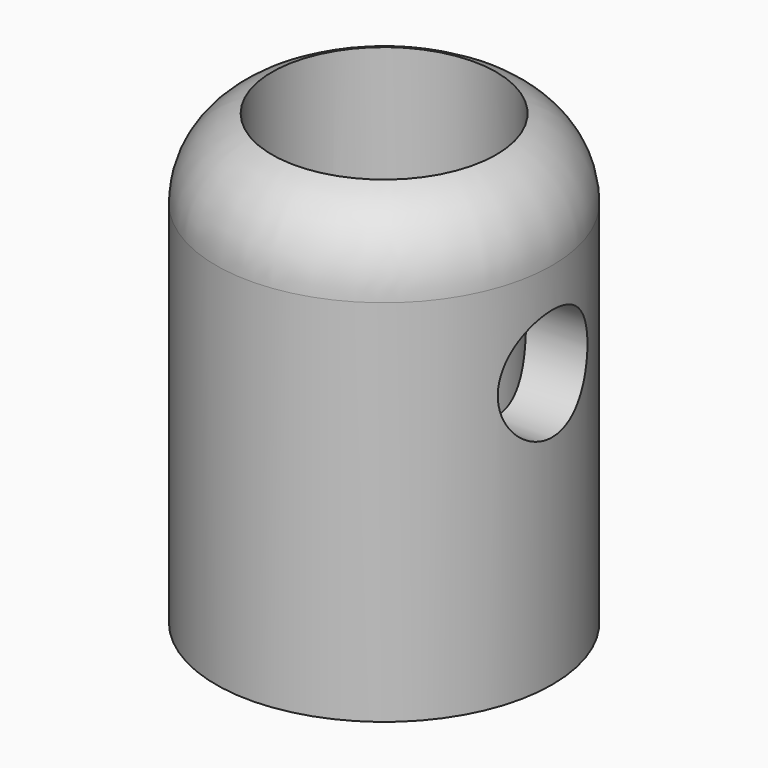
from build123d import *

# Parameters (mm, degrees)
F0_R     = 6
F1_DEPTH = 16
F2_R     = 2
F3_DEPTH = 12.5
F4_R     = 4
F5_DEPTH = 12


# Not quite as in the source:
# - a fillet or chamfer that OpenCascade refuses, or shapes differently, is made with other operations: its cross-section is extruded or revolved along the edge and cut away or added


with BuildPart() as f1:
    # F0 (on Top) → F1 (new body)
    with BuildSketch(Plane.XY):
        Circle(F0_R)
    extrude(amount=F1_DEPTH)

    # F2 (on Right) → F3 (cut, symmetric)
    with BuildSketch(Plane.YZ):
        with Locations((0, 9.7745376602)):
            Circle(F2_R)
    extrude(amount=F3_DEPTH, both=True, mode=Mode.SUBTRACT)

    # F4 (on face) → F5 (cut)
    with BuildSketch(Plane.XY.offset(16)):
        Circle(F4_R)
    extrude(amount=-F5_DEPTH, mode=Mode.SUBTRACT)

    # F6: fillet of radius 3 on 1 edges, made by hand

    # F6_s1 → F6_t2 (revolve, cut)
    with BuildSketch(Plane.XZ):
        with BuildLine():
            ThreePointArc((6, 13.1715728753), (5.4494897428, 14.9036236828), (4, 16))
            Line((4, 16), (6, 16))
            Line((6, 16), (6, 13.1715728753))
        make_face()
    revolve(axis=Axis((0, 0, 16), (0, 0, 1)), mode=Mode.SUBTRACT)


solid = f1.part
